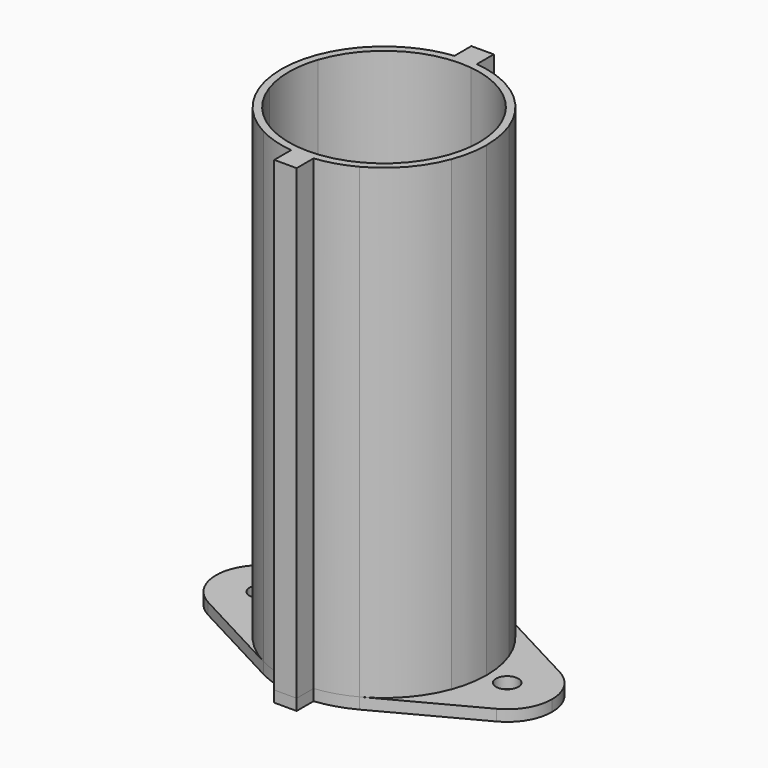
from build123d import *
from build123d import SkipClean  # not in build123d's __all__

# Parameters (mm, degrees)
F0_R     = 3
F1_DEPTH = 3
F2_DEPTH = 125


# Not quite as in the source:
# - a feature names something its author has since deleted; it is built from what else it names


with BuildPart() as f1:
    # F0 (on Top) → F1 (new body)
    with BuildSketch(Plane.XY):
        with BuildLine():
            ThreePointArc((12.9166666896, 24.2777618744), (20.6949130465, 18.1099578685), (25.7765151515, 9.5823413967))
            ThreePointArc((25.7765151515, 9.5823413967), (32.0589540907, 11.9630444535), (38.6363637791, 10.5939323837))
            Line((38.6363637791, 10.5939323837), (12.9166666896, 24.2777618744))
        make_face()
        with BuildLine():
            ThreePointArc((25.7765151515, 9.5823413967), (27.0656993875, 4.8680506023), (27.5, 0))
            ThreePointArc((27.5, 0), (27.0656993875, -4.8680506023), (25.7765151515, -9.5823413967))
            ThreePointArc((25.7765151515, -9.5823413967), (32.0589541175, -11.9630444556), (38.6363638266, -10.5939323584))
            ThreePointArc((38.6363638266, -10.5939323584), (43.2867965353, -6.1791437142), (45, 0))
            ThreePointArc((45, 0), (43.2867965215, 6.1791437372), (38.6363637791, 10.5939323837))
            ThreePointArc((38.6363637791, 10.5939323837), (32.0589540907, 11.9630444535), (25.7765151515, 9.5823413967))
        make_face()
        with Locations((33, 0)):
            Circle(F0_R, mode=Mode.SUBTRACT)
        with BuildLine():
            ThreePointArc((25.7765151515, -9.5823413967), (27.0656993875, -4.8680506023), (27.5, 0))
            ThreePointArc((27.5, 0), (27.0656993875, 4.8680506023), (25.7765151515, 9.5823413967))
            ThreePointArc((25.7765151515, 9.5823413967), (24.9405426226, 8.8907337595), (24.1704545455, 8.1264461523))
            ThreePointArc((24.1704545455, 8.1264461523), (25.1654186425, 4.117244776), (25.5, 0))
            ThreePointArc((25.5, 0), (25.1654186425, -4.117244776), (24.1704545455, -8.1264461523))
            ThreePointArc((24.1704545455, -8.1264461523), (24.9405426226, -8.8907337595), (25.7765151515, -9.5823413967))
        make_face()
        with BuildLine():
            ThreePointArc((-3, 27.3358738657), (0, 27.5), (3, 27.3358738657))
            Line((3, 27.3358738657), (3, 33))
            Line((3, 33), (-3, 33))
            Line((-3, 33), (-3, 27.3358738657))
        make_face()
        with BuildLine():
            ThreePointArc((38.6363638266, -10.5939323584), (32.0589541175, -11.9630444556), (25.7765151515, -9.5823413967))
            ThreePointArc((25.7765151515, -9.5823413967), (20.6949131964, -18.1099576972), (12.9166670915, -24.2777616606))
            Line((12.9166670915, -24.2777616606), (38.6363638266, -10.5939323584))
        make_face()
        with BuildLine():
            ThreePointArc((-25.7765151515, 9.5823413967), (-20.6949129227, 18.1099580099), (-12.9166663578, 24.2777620509))
            Line((-12.9166663578, 24.2777620509), (-38.636363452, 10.5939325577))
            ThreePointArc((-38.636363452, 10.5939325577), (-32.058953906, 11.963044439), (-25.7765151515, 9.5823413967))
        make_face()
        with BuildLine():
            ThreePointArc((-25.7765151515, -9.5823413967), (-27.5, 0), (-25.7765151515, 9.5823413967))
            ThreePointArc((-25.7765151515, 9.5823413967), (-32.058953906, 11.963044439), (-38.636363452, 10.5939325577))
            ThreePointArc((-38.636363452, 10.5939325577), (-45, 1.496e-07), (-38.6363637162, -10.5939324171))
            ThreePointArc((-38.6363637162, -10.5939324171), (-32.0589540552, -11.9630444507), (-25.7765151515, -9.5823413967))
        make_face()
        with Locations((-33, 0)):
            Circle(F0_R, mode=Mode.SUBTRACT)
        with BuildLine():
            ThreePointArc((-24.1704545455, -8.1264461523), (-25.5, 0), (-24.1704545455, 8.1264461523))
            ThreePointArc((-24.1704545455, 8.1264461523), (-24.9405426226, 8.8907337595), (-25.7765151515, 9.5823413967))
            ThreePointArc((-25.7765151515, 9.5823413967), (-27.5, 0), (-25.7765151515, -9.5823413967))
            ThreePointArc((-25.7765151515, -9.5823413967), (-24.9405426226, -8.8907337595), (-24.1704545455, -8.1264461523))
        make_face()
        with BuildLine():
            Line((-38.6363637162, -10.5939324171), (-12.9166665881, -24.2777619284))
            ThreePointArc((-12.9166665881, -24.2777619284), (-20.6949130086, -18.1099579118), (-25.7765151515, -9.5823413967))
            ThreePointArc((-25.7765151515, -9.5823413967), (-32.0589540552, -11.9630444507), (-38.6363637162, -10.5939324171))
        make_face()
        with BuildLine():
            Line((3, 25.3229145242), (3, 27.3358738657))
            ThreePointArc((3, 27.3358738657), (0, 27.5), (-3, 27.3358738657))
            Line((-3, 27.3358738657), (-3, 25.3229145242))
            ThreePointArc((-3, 25.3229145242), (0, 25.5), (3, 25.3229145242))
        make_face()
        with BuildLine():
            ThreePointArc((24.1704545455, 8.1264461523), (24.9405426226, 8.8907337595), (25.7765151515, 9.5823413967))
            ThreePointArc((25.7765151515, 9.5823413967), (20.6949130465, 18.1099578685), (12.9166666896, 24.2777618744))
            ThreePointArc((12.9166666896, 24.2777618744), (8.1038930067, 26.2788302277), (3, 27.3358738657))
            Line((3, 27.3358738657), (3, 25.3229145242))
            ThreePointArc((3, 25.3229145242), (16.0775629735, 19.7929777657), (24.1704545455, 8.1264461523))
        make_face()
        with BuildLine():
            Line((-3, 25.3229145242), (-3, 27.3358738657))
            ThreePointArc((-3, 27.3358738657), (-8.1038928272, 26.2788302831), (-12.9166663578, 24.2777620509))
            ThreePointArc((-12.9166663578, 24.2777620509), (-20.6949129227, 18.1099580099), (-25.7765151515, 9.5823413967))
            ThreePointArc((-25.7765151515, 9.5823413967), (-24.9405426226, 8.8907337595), (-24.1704545455, 8.1264461523))
            ThreePointArc((-24.1704545455, 8.1264461523), (-16.0775629735, 19.7929777657), (-3, 25.3229145242))
        make_face()
        with BuildLine():
            ThreePointArc((-3, -27.3358738657), (0, -27.5), (3, -27.3358738657))
            Line((3, -27.3358738657), (3, -25.3229145242))
            ThreePointArc((3, -25.3229145242), (0, -25.5), (-3, -25.3229145242))
            Line((-3, -25.3229145242), (-3, -27.3358738657))
        make_face()
        with BuildLine():
            Line((3, -33), (3, -27.3358738657))
            ThreePointArc((3, -27.3358738657), (0, -27.5), (-3, -27.3358738657))
            Line((-3, -27.3358738657), (-3, -33))
            Line((-3, -33), (3, -33))
        make_face()
        with BuildLine():
            ThreePointArc((12.9166670915, -24.2777616606), (20.6949131964, -18.1099576972), (25.7765151515, -9.5823413967))
            ThreePointArc((25.7765151515, -9.5823413967), (24.9405426226, -8.8907337595), (24.1704545455, -8.1264461523))
            ThreePointArc((24.1704545455, -8.1264461523), (16.0775629735, -19.7929777657), (3, -25.3229145242))
            Line((3, -25.3229145242), (3, -27.3358738657))
            ThreePointArc((3, -27.3358738657), (8.1038932243, -26.2788301606), (12.9166670915, -24.2777616606))
        make_face()
        with BuildLine():
            ThreePointArc((-12.9166665881, -24.2777619284), (-8.1038929518, -26.2788302446), (-3, -27.3358738657))
            Line((-3, -27.3358738657), (-3, -25.3229145242))
            ThreePointArc((-3, -25.3229145242), (-16.0775629735, -19.7929777657), (-24.1704545455, -8.1264461523))
            ThreePointArc((-24.1704545455, -8.1264461523), (-24.9405426226, -8.8907337595), (-25.7765151515, -9.5823413967))
            ThreePointArc((-25.7765151515, -9.5823413967), (-20.6949130086, -18.1099579118), (-12.9166665881, -24.2777619284))
        make_face()
    extrude(amount=-F1_DEPTH)

    # F0 (on Top) → F2 (join)
    with BuildSketch(Plane.XY):
        with BuildLine():
            Line((-3, 25.3229145242), (-3, 27.3358738657))
            ThreePointArc((-3, 27.3358738657), (-8.1038928272, 26.2788302831), (-12.9166663578, 24.2777620509))
            ThreePointArc((-12.9166663578, 24.2777620509), (-20.6949129227, 18.1099580099), (-25.7765151515, 9.5823413967))
            ThreePointArc((-25.7765151515, 9.5823413967), (-24.9405426226, 8.8907337595), (-24.1704545455, 8.1264461523))
            ThreePointArc((-24.1704545455, 8.1264461523), (-16.0775629735, 19.7929777657), (-3, 25.3229145242))
        make_face()
        with BuildLine():
            ThreePointArc((-3, 27.3358738657), (0, 27.5), (3, 27.3358738657))
            Line((3, 27.3358738657), (3, 33))
            Line((3, 33), (-3, 33))
            Line((-3, 33), (-3, 27.3358738657))
        make_face()
        with BuildLine():
            Line((3, 25.3229145242), (3, 27.3358738657))
            ThreePointArc((3, 27.3358738657), (0, 27.5), (-3, 27.3358738657))
            Line((-3, 27.3358738657), (-3, 25.3229145242))
            ThreePointArc((-3, 25.3229145242), (0, 25.5), (3, 25.3229145242))
        make_face()
        with BuildLine():
            ThreePointArc((24.1704545455, 8.1264461523), (24.9405426226, 8.8907337595), (25.7765151515, 9.5823413967))
            ThreePointArc((25.7765151515, 9.5823413967), (20.6949130465, 18.1099578685), (12.9166666896, 24.2777618744))
            ThreePointArc((12.9166666896, 24.2777618744), (8.1038930067, 26.2788302277), (3, 27.3358738657))
            Line((3, 27.3358738657), (3, 25.3229145242))
            ThreePointArc((3, 25.3229145242), (16.0775629735, 19.7929777657), (24.1704545455, 8.1264461523))
        make_face()
        with BuildLine():
            Line((3, -33), (3, -27.3358738657))
            ThreePointArc((3, -27.3358738657), (0, -27.5), (-3, -27.3358738657))
            Line((-3, -27.3358738657), (-3, -33))
            Line((-3, -33), (3, -33))
        make_face()
        with BuildLine():
            ThreePointArc((-24.1704545455, -8.1264461523), (-25.5, 0), (-24.1704545455, 8.1264461523))
            ThreePointArc((-24.1704545455, 8.1264461523), (-24.9405426226, 8.8907337595), (-25.7765151515, 9.5823413967))
            ThreePointArc((-25.7765151515, 9.5823413967), (-27.5, 0), (-25.7765151515, -9.5823413967))
            ThreePointArc((-25.7765151515, -9.5823413967), (-24.9405426226, -8.8907337595), (-24.1704545455, -8.1264461523))
        make_face()
        with BuildLine():
            ThreePointArc((25.7765151515, -9.5823413967), (27.0656993875, -4.8680506023), (27.5, 0))
            ThreePointArc((27.5, 0), (27.0656993875, 4.8680506023), (25.7765151515, 9.5823413967))
            ThreePointArc((25.7765151515, 9.5823413967), (24.9405426226, 8.8907337595), (24.1704545455, 8.1264461523))
            ThreePointArc((24.1704545455, 8.1264461523), (25.1654186425, 4.117244776), (25.5, 0))
            ThreePointArc((25.5, 0), (25.1654186425, -4.117244776), (24.1704545455, -8.1264461523))
            ThreePointArc((24.1704545455, -8.1264461523), (24.9405426226, -8.8907337595), (25.7765151515, -9.5823413967))
        make_face()
        with BuildLine():
            ThreePointArc((-3, -27.3358738657), (0, -27.5), (3, -27.3358738657))
            Line((3, -27.3358738657), (3, -25.3229145242))
            ThreePointArc((3, -25.3229145242), (0, -25.5), (-3, -25.3229145242))
            Line((-3, -25.3229145242), (-3, -27.3358738657))
        make_face()
        with BuildLine():
            ThreePointArc((-12.9166665881, -24.2777619284), (-8.1038929518, -26.2788302446), (-3, -27.3358738657))
            Line((-3, -27.3358738657), (-3, -25.3229145242))
            ThreePointArc((-3, -25.3229145242), (-16.0775629735, -19.7929777657), (-24.1704545455, -8.1264461523))
            ThreePointArc((-24.1704545455, -8.1264461523), (-24.9405426226, -8.8907337595), (-25.7765151515, -9.5823413967))
            ThreePointArc((-25.7765151515, -9.5823413967), (-20.6949130086, -18.1099579118), (-12.9166665881, -24.2777619284))
        make_face()
        with BuildLine():
            ThreePointArc((12.9166670915, -24.2777616606), (20.6949131964, -18.1099576972), (25.7765151515, -9.5823413967))
            ThreePointArc((25.7765151515, -9.5823413967), (24.9405426226, -8.8907337595), (24.1704545455, -8.1264461523))
            ThreePointArc((24.1704545455, -8.1264461523), (16.0775629735, -19.7929777657), (3, -25.3229145242))
            Line((3, -25.3229145242), (3, -27.3358738657))
            ThreePointArc((3, -27.3358738657), (8.1038932243, -26.2788301606), (12.9166670915, -24.2777616606))
        make_face()
    with SkipClean():  # cleaning this boolean's faces spoils the solid; the shape is the same uncleaned
        extrude(amount=F2_DEPTH)


solid = f1.part
